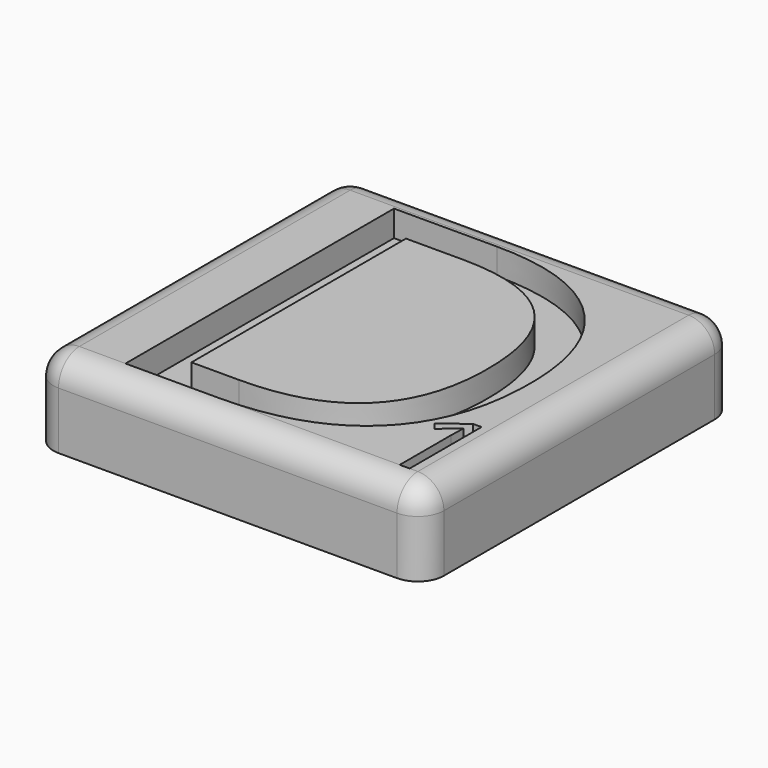
from build123d import *

# Parameters (mm, degrees)
F0_W         = 19.05
F0_H         = 19.05
F1_DEPTH     = 4.064
F2_R         = 1.27
F3_TEXT_SIZE = 22.9305555556
F4_DEPTH     = 1.27
F5_TEXT_SIZE = 6.1366553416
F6_DEPTH     = 1.27


# Not quite as in the source:
# - Text() gives the source's letters only with a copy of the font that has no kerning and outlines rounded to 1/6400 em; it was checked with that copy


with BuildPart() as f1:
    # F0 (on Top) → F1 (new body)
    with BuildSketch(Plane.XY):
        with Locations((9.525, 9.525)):
            Rectangle(F0_W, F0_H)
    extrude(amount=F1_DEPTH)

    # F2
    f2_edges = [f1.edges().sort_by_distance(p)[0] for p in [
        (19.05, 0, 2.032),
        (19.05, 9.525, 4.064),
        (9.525, 0, 4.064),
        (0, 0, 2.032),
        (0, 9.525, 4.064),
        (19.05, 19.05, 2.032),
        (9.525, 19.05, 4.064),
        (0, 19.05, 2.032),
    ]]
    fillet(f2_edges, radius=F2_R)

    # F3 (on face) → F4 (cut)
    with BuildSketch(Plane.XY.offset(4.064)):
        with Locations((1.27, 1.27)):
            Text('D', F3_TEXT_SIZE, font='Open Sans', text_align=(TextAlign.LEFT, TextAlign.BOTTOM))
    extrude(amount=-F4_DEPTH, mode=Mode.SUBTRACT)

    # F5 (on face) → F6 (cut)
    with BuildSketch(Plane.XY.offset(4.064)):
        with Locations((15.24, 1.27)):
            Text('1', F5_TEXT_SIZE, font='Open Sans', text_align=(TextAlign.LEFT, TextAlign.BOTTOM))
    extrude(amount=-F6_DEPTH, mode=Mode.SUBTRACT)


solid = f1.part
